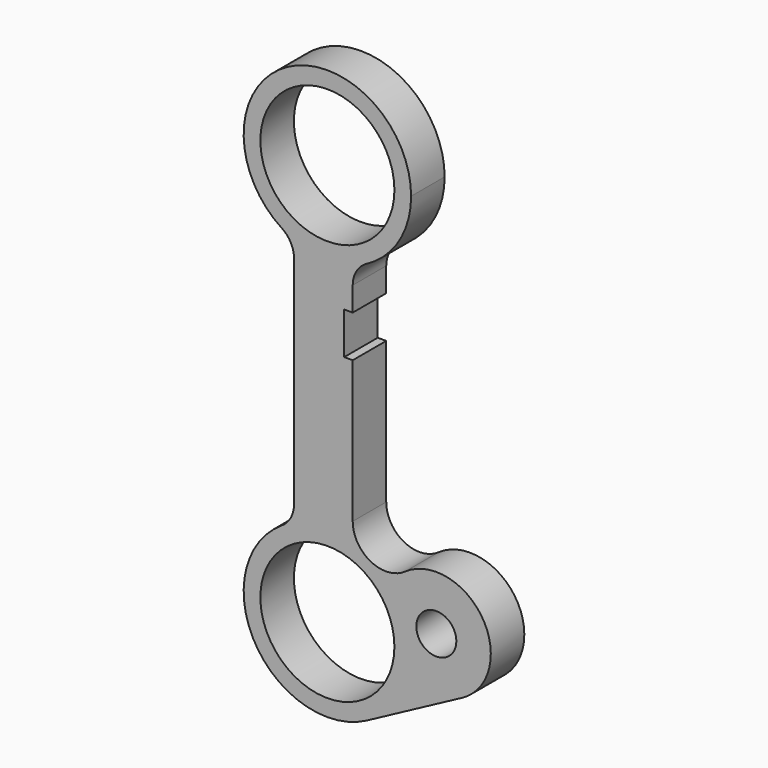
from build123d import *

# Parameters (mm, degrees)
F1_DEPTH = 5.0038
F2_R     = 3.175
F3_R     = 8.001
F4_DEPTH = 5.0038
F5_W     = 1.016
F5_H     = 5.0038
F6_DEPTH = 5.0038
F7_R     = 2.3876
F8_DEPTH = 5.0038


with BuildPart() as f1:
    # F0 (on Front) → F1 (new body)
    with BuildSketch(Plane.XZ):
        with BuildLine():
            ThreePointArc((9.9949, 48.006), (-5.4790676118, 56.3652968673), (-3.9878, 38.841095354))
            ThreePointArc((-3.9878, 38.841095354), (-0.5154258333, 38.0243988148), (3.0226, 38.4790951905))
            ThreePointArc((3.0226, 38.4790951905), (8.0656249215, 42.1031430108), (9.9949, 48.006))
        make_face()
        with BuildLine():
            Line((-3.9878, 38.841095354), (-3.9878, 9.164904646))
            ThreePointArc((-3.9878, 9.164904646), (-8.9961822265, -4.3550810966), (4.7152403545, -8.8127484027))
            Line((4.7152403545, -8.8127484027), (16.0724023653, -2.7361255174))
            ThreePointArc((16.0724023653, -2.7361255174), (18.5431093303, 6.4043007502), (9.270553305, 8.3204140086))
            ThreePointArc((9.270553305, 8.3204140086), (5.1603136206, 8.0483265237), (3.0226, 11.5694459962))
            Line((3.0226, 11.5694459962), (3.0226, 38.4790951905))
            ThreePointArc((3.0226, 38.4790951905), (-0.5154258333, 38.0243988148), (-3.9878, 38.841095354))
        make_face()
    extrude(amount=F1_DEPTH)

    # F2
    f2_edges = [f1.edges().sort_by_distance(p)[0] for p in [
        (-3.9878, -2.5019, 38.841095),
        (3.0226, -2.5019, 38.479095),
        (-3.9878, -2.5019, 9.164905),
    ]]
    fillet(f2_edges, radius=F2_R)

    # F3 (on face) → F4 (cut)
    with BuildSketch(Plane.XZ.offset(5.0038)):
        with Locations((0, 48.006)):
            Circle(F3_R)
        Circle(F3_R)
    extrude(amount=-F4_DEPTH, mode=Mode.SUBTRACT)

    # F5 (on face) → F6 (cut)
    with BuildSketch(Plane.XZ.offset(5.0038)):
        with Locations((2.5146, 31.0007)):
            Rectangle(F5_W, F5_H)
    extrude(amount=-F6_DEPTH, mode=Mode.SUBTRACT)

    # F7 (on face) → F8 (cut)
    with BuildSketch(Plane.XZ.offset(5.0038)):
        with Locations((13.0048, 2.9972)):
            Circle(F7_R)
    extrude(amount=-F8_DEPTH, mode=Mode.SUBTRACT)


solid = f1.part
